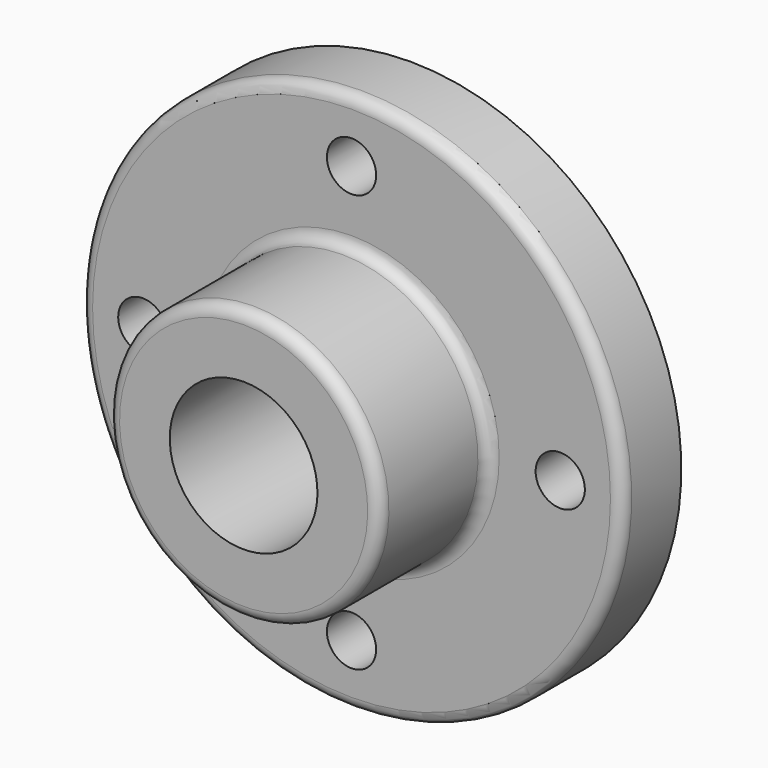
from build123d import *

# Parameters (mm, degrees)
F2_R            = 6.35
F3_DEPTH        = 19.051
F3_COPIES_COUNT = 4
F4_R            = 3.048


# Not quite as in the source:
# - a pattern or mirror of a feature is missing from the dataset's text; its kind, count and spacing are read off the source's solid


with BuildPart() as f1:
    # F0 (on Right) → F1 (revolve)
    with BuildSketch(Plane.YZ):
        Polygon((-53.848, 19.05), (0, 19.05), (0, 69.85), (-19.05, 69.85), (-19.05, 35.052), (-53.848, 35.052), align=None)
    revolve(axis=Axis((0, -55.1984038566, 0), (0, -1, 0)))

    # F2 (on face) → F3 (cut, through all)
    with BuildSketch(Plane.XZ.offset(19.05)):
        with Locations((0, 53.848)):
            Circle(F2_R)
    f3 = extrude(amount=-F3_DEPTH, mode=Mode.SUBTRACT)

    # F3_copies: F3 ×4 about axis
    f3_copies_axis = Axis((0, 0, 0), (0, 1, 0))
    for i in range(1, F3_COPIES_COUNT):
        add(f3.rotate(f3_copies_axis, i * 360 / F3_COPIES_COUNT), mode=Mode.SUBTRACT)

    # F4
    f4_edges = [f1.edges().sort_by_distance(p)[0] for p in [
        (0, -19.05, -69.85),
        (0, -19.05, -35.052),
        (0, -53.848, -35.052),
    ]]
    fillet(f4_edges, radius=F4_R)


solid = f1.part
